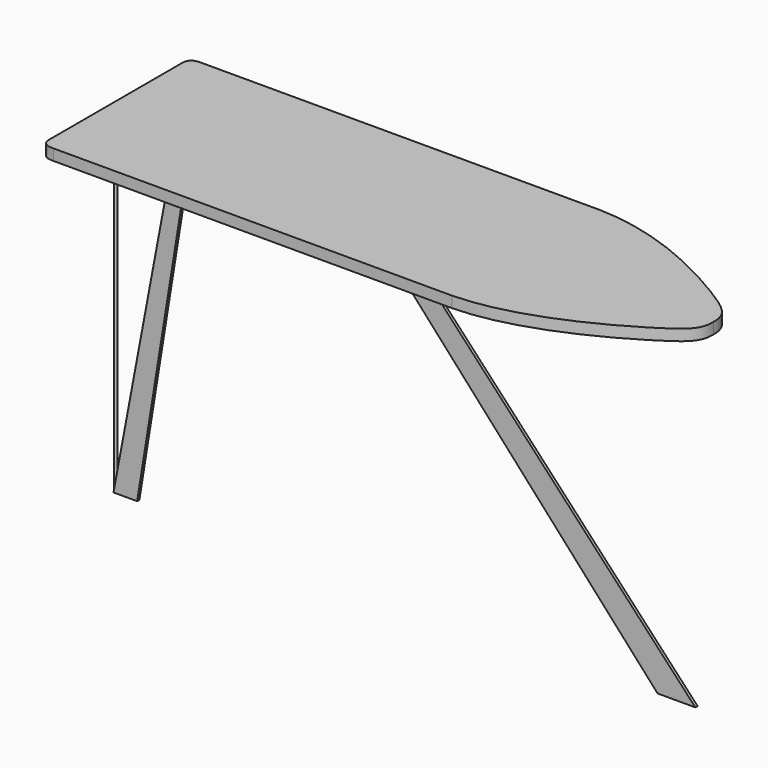
from build123d import *

# Parameters (mm, degrees)
F1_R     = 3.175
F2_DEPTH = 762
F3_DEPTH = 6.35
F5_DEPTH = 25.4


with BuildPart() as f2:
    # F1 (on Top) → F2 (new body)
    with BuildSketch(Plane.XY):
        Circle(F1_R)
    extrude(amount=F2_DEPTH)


with BuildPart() as f3:
    # F0 (on Front) → F3 (new body)
    with BuildSketch(Plane.XZ):
        Polygon((1247.8656768799, 0), (1334.6340656281, 0), (625.6737112999, 762), (562.1847510338, 762), align=None)
    extrude(amount=F3_DEPTH)



with BuildPart() as f3b:
    # F0 (on Front) → F3, piece 2 (new body)
    with BuildSketch(Plane.XZ):
        Polygon((143.1574821472, 762), (0, 0), (54.2729124427, 0), (177.0182698965, 762), align=None)
    extrude(amount=F3_DEPTH)


with BuildPart() as f3_1:
    add(f3.part)

    add(f3b.part)  # F5 merges F3b
    # F4 (on face) → F5 (join)
    with BuildSketch(Plane.XY.offset(762)):
        with BuildLine():
            Line((0, 190.5), (0, 0))
            Line((0, 0), (0, -190.5))
            add(Edge.make_bspline(
                [(0, -190.5), (0, -208.3280831575), (11.9508374482, -212.820827961), (27.0897336304, -212.4256193638)],
                knots=[0, 0, 0, 0, 34.8509175296, 34.8509175296, 34.8509175296, 34.8509175296], degree=3))
            Line((27.0897336304, -212.4256193638), (941.4897336304, -212.4256193638))
            add(Edge.make_bspline(
                [(941.4897336304, -212.4256193638), (1084.1052532196, -209.4828337431), (1306.4068704852, -88.0603993583), (1372.2732067108, -35.1411737502), (1370.5102205276, 0)],
                knots=[0, 0, 0, 0, 0.6669321304, 1, 1, 1, 1], degree=3))
            add(Edge.make_bspline(
                [(941.4897336304, 212.4256193638), (1084.1052532196, 209.4828337431), (1306.4068704852, 88.0603993583), (1372.2732067108, 35.1411737502), (1370.5102205276, 0)],
                knots=[0, 0, 0, 0, 0.6669321304, 1, 1, 1, 1], degree=3))
            Line((941.4897336304, 212.4256193638), (27.0897336304, 212.4256193638))
            add(Edge.make_bspline(
                [(0, 190.5), (0, 208.3280831575), (11.9508374482, 212.820827961), (27.0897336304, 212.4256193638)],
                knots=[0, 0, 0, 0, 34.8509175296, 34.8509175296, 34.8509175296, 34.8509175296], degree=3))
        make_face()
    extrude(amount=F5_DEPTH)


solid = Compound([f2.part, f3_1.part])
